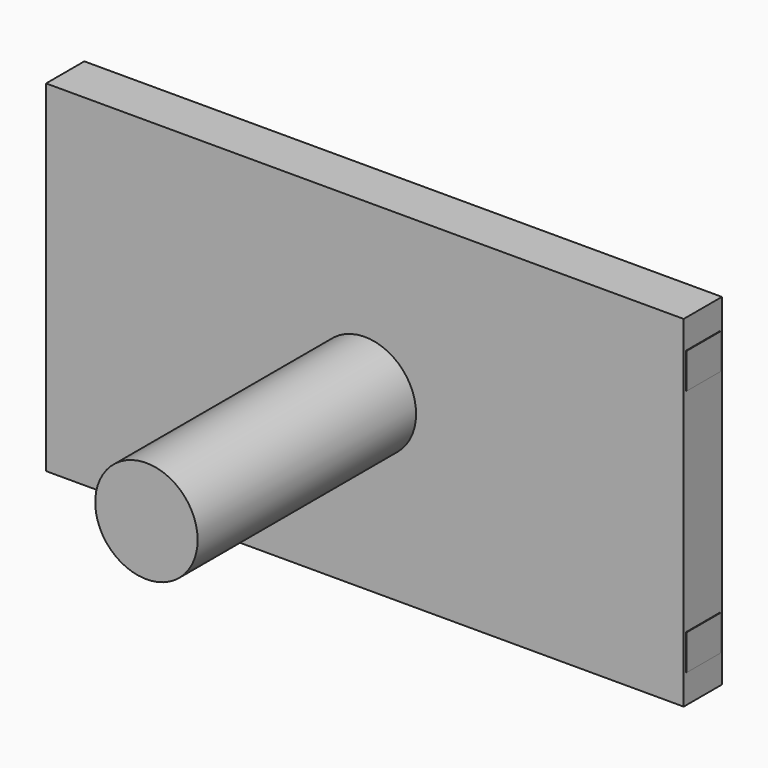
from build123d import *

# Parameters (mm, degrees)
F0_W     = 934
F0_H     = 500
F1_DEPTH = 70
F2_R     = 75
F3_DEPTH = 400
F4_W     = 62
F4_H     = 51.8
F5_DEPTH = 1


# Not quite as in the source:
# - a pattern or mirror of a feature is missing from the dataset's text; its kind, count and spacing are read off the source's solid


with BuildPart() as f1:
    # F0 (on Front) → F1 (new body)
    with BuildSketch(Plane.XZ):
        Rectangle(F0_W, F0_H)
    extrude(amount=F1_DEPTH)

    # F2 (on face) → F3 (join)
    with BuildSketch(Plane.XZ.offset(70)):
        Circle(F2_R)
    extrude(amount=F3_DEPTH)

    # F4 (on face) → F5 (join)
    with BuildSketch(Plane.YZ.offset(467)):
        with Locations((-35, 181.5)):
            Rectangle(F4_W, F4_H)
        with Locations((-35, -181.5)):
            Rectangle(F4_W, F4_H)
    f5 = extrude(amount=F5_DEPTH)

    # F5_copies: F5 across plane
    add(f5.mirror(Plane(origin=(0, 0, 0), x_dir=(0, 0, -1), z_dir=(-1, 0, 0))))


solid = f1.part
